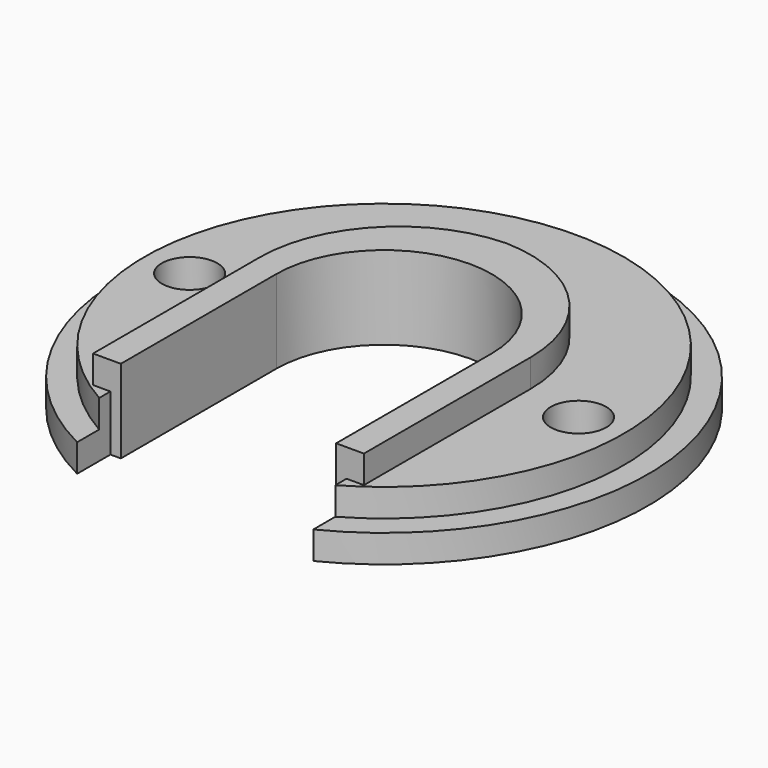
from build123d import *

# Parameters (mm, degrees)
F0_R        = 19
F1_DEPTH    = 2
F2_R        = 17.25
F3_DEPTH    = 2
F5_DEPTH    = 25
F7_DEPTH    = 6
F8_T1_DEPTH = 27
F9_R        = 2
F10_DEPTH   = 25
F11_R       = 2
F12_DEPTH   = 25
F13_R       = 2
F14_DEPTH   = 25


# Not quite as in the source:
# - a fillet or chamfer that OpenCascade refuses, or shapes differently, is made with other operations: its cross-section is extruded or revolved along the edge and cut away or added


with BuildPart() as f1:
    # F0 (on Top) → F1 (new body)
    with BuildSketch(Plane.XY):
        Circle(F0_R)
    extrude(amount=F1_DEPTH)

    # F2 (on face) → F3 (join)
    with BuildSketch(Plane.XY.offset(2)):
        Circle(F2_R)
    extrude(amount=F3_DEPTH)

    # F4 (on face) → F5 (cut)
    with BuildSketch(Plane.XY.offset(4)):
        with BuildLine():
            Line((0, 0), (8.5, 0))
            ThreePointArc((8.5, 0), (0, 8.5), (-8.5, 0))
            Line((-8.5, 0), (0, 0))
        make_face()
        with BuildLine():
            ThreePointArc((-8.5, 0), (0, -8.5), (8.5, 0))
            Line((8.5, 0), (0, 0))
            Line((0, 0), (-8.5, 0))
        make_face()
        with BuildLine():
            Line((8.5, -31.9736860693), (8.5, -15.0104130523))
            ThreePointArc((8.5, -15.0104130523), (0, -17.25), (-8.5, -15.0104130523))
            Line((-8.5, -15.0104130523), (-8.5, -31.0855284333))
            Line((-8.5, -31.0855284333), (8.5, -31.9736860693))
        make_face()
        with BuildLine():
            Line((8.5, -15.0104130523), (8.5, 0))
            ThreePointArc((8.5, 0), (0, -8.5), (-8.5, 0))
            Line((-8.5, 0), (-8.5, -15.0104130523))
            ThreePointArc((-8.5, -15.0104130523), (0, -17.25), (8.5, -15.0104130523))
        make_face()
    extrude(amount=-F5_DEPTH, mode=Mode.SUBTRACT)

    # F6 (on Top) → F7 (join)
    with BuildSketch(Plane.XY):
        with BuildLine():
            ThreePointArc((-7.75, 0), (0, 7.75), (7.75, 0))
            Line((7.75, 0), (7.75, -14))
            Line((7.75, -14), (9.75, -14))
            Line((9.75, -14), (9.75, 11))
            Line((9.75, 11), (-9.75, 11))
            Line((-9.75, 11), (-9.75, -14))
            Line((-9.75, -14), (-7.75, -14))
            Line((-7.75, -14), (-7.75, 0))
        make_face()
    extrude(amount=F7_DEPTH)

    # F8: fillet of radius 10 on 2 edges, made by hand

    # F8_s2 → F8_t1 (cut)
    with BuildSketch(Plane.XY.offset(4)):
        with BuildLine():
            ThreePointArc((9.75, 1), (6.8210678119, 8.0710678119), (-0.25, 11))
            Line((-0.25, 11), (9.75, 11))
            Line((9.75, 11), (9.75, 1))
        make_face()
        with BuildLine():
            ThreePointArc((0.25, 11), (-6.8210678119, 8.0710678119), (-9.75, 1))
            Line((-9.75, 1), (-9.75, 11))
            Line((-9.75, 11), (0.25, 11))
        make_face()
    extrude(amount=F8_T1_DEPTH, mode=Mode.SUBTRACT)

    # F9 (on face) → F10 (cut)
    with BuildSketch(Plane.XY.offset(2)):
        with Locations((14, 0)):
            Circle(F9_R)
        with BuildLine():
            ThreePointArc((-16, 0), (-14, -2), (-12, 0))
            ThreePointArc((-12, 0), (-14, 2), (-16, 0))
        make_face()
    extrude(amount=-F10_DEPTH, mode=Mode.SUBTRACT)

    # F11 (on face) → F12 (cut)
    with BuildSketch(Plane(origin=(0, 0, 2), x_dir=(1, 0, 0), z_dir=(0, 0, -1))):
        with Locations((-14, 0)):
            Circle(F11_R)
    extrude(amount=-F12_DEPTH, mode=Mode.SUBTRACT)

    # F13 (on face) → F14 (cut)
    with BuildSketch(Plane(origin=(0, 0, 2), x_dir=(1, 0, 0), z_dir=(0, 0, -1))):
        with Locations((14, 0)):
            Circle(F13_R)
    extrude(amount=-F14_DEPTH, mode=Mode.SUBTRACT)


solid = f1.part
